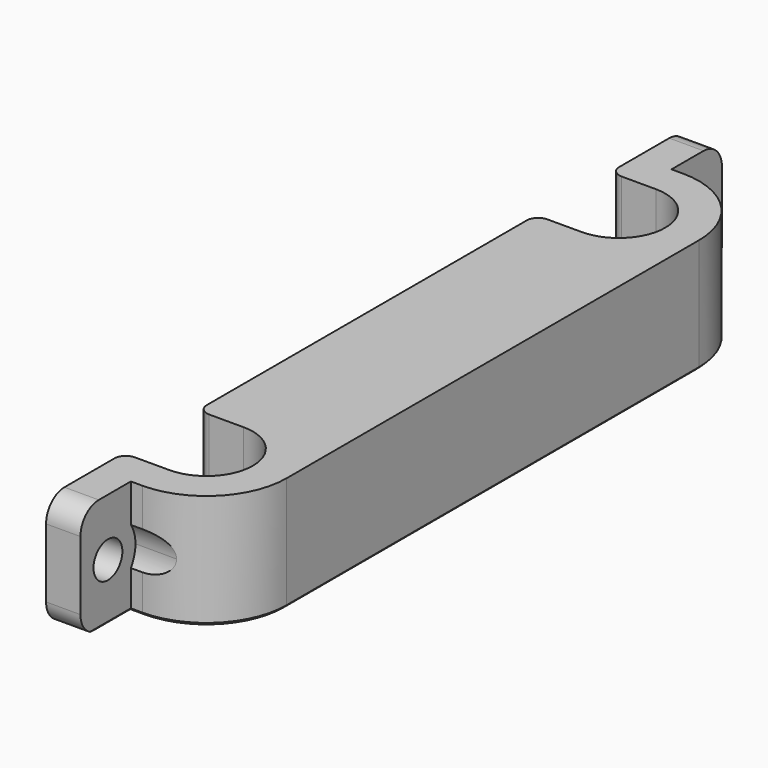
from build123d import *

# Parameters (mm, degrees)
F1_DEPTH     = 5
F2_R         = 1
F3_R         = 1.575
F4_DEPTH     = 3
F3_R_2       = 3
F5_DEPTH     = 8.001
F6_R         = 2
F7_T1_DEPTH  = 6.5429652699
F7_T3_DEPTH  = 3
F7_T5_DEPTH  = 45
F7_T7_DEPTH  = 34.9
F7_T9_DEPTH  = 6.5429652699
F7_T12_ANGLE = 90
F7_T16_DEPTH = 5.2358860169
F7_T21_DEPTH = 1.642920747
F7_T24_ANGLE = 180
F7_T26_ANGLE = 90
F7_T28_ANGLE = 90
F7_T30_ANGLE = 90
F7_T34_DEPTH = 1.642920747
F7_T37_ANGLE = 90
F7_T41_DEPTH = 5.2358860169
F7_T44_ANGLE = 180
F7_T46_ANGLE = 90


# Not quite as in the source:
# - a fillet or chamfer that OpenCascade refuses, or shapes differently, is made with other operations: its cross-section is extruded or revolved along the edge and cut away or added


with BuildPart() as f1:
    # F0 (on Top) → F1 (new body, symmetric)
    with BuildSketch(Plane.XY):
        with BuildLine():
            Line((-4, 26.55), (0, 26.55))
            ThreePointArc((0, 26.55), (4.05, 22.5), (0, 18.45))
            Line((0, 18.45), (-4, 18.45))
            Line((-4, 18.45), (-4, 0))
            Line((-4, 0), (-4, -18.45))
            Line((-4, -18.45), (0, -18.45))
            ThreePointArc((0, -18.45), (4.05, -22.5), (0, -26.55))
            Line((0, -26.55), (-4, -26.55))
            Line((-4, -26.55), (-4, -35))
            Line((-4, -35), (-1, -35))
            Line((-1, -35), (-1, -29.5))
            Line((-1, -29.5), (0, -29.5))
            ThreePointArc((0, -29.5), (4.9497474683, -27.4497474683), (7, -22.5))
            Line((7, -22.5), (7, 0))
            Line((7, 0), (7, 22.5))
            ThreePointArc((7, 22.5), (4.9497474683, 27.4497474683), (0, 29.5))
            Line((0, 29.5), (-1, 29.5))
            Line((-1, 29.5), (-1, 35))
            Line((-1, 35), (-4, 35))
            Line((-4, 35), (-4, 26.55))
        make_face()
    extrude(amount=F1_DEPTH, both=True)

    # F2
    f2_edges = [f1.edges().sort_by_distance(p)[0] for p in [
        (-4, 26.55, 0),
        (-4, 18.45, 0),
        (-4, -26.55, 0),
        (-4, -18.45, 0),
    ]]
    fillet(f2_edges, radius=F2_R)

    # F3 (on face) → F4 (cut, through all)
    with BuildSketch(Plane.YZ.offset(-1)):
        with Locations((32, 0)):
            Circle(F3_R)
        with Locations((-32, 0)):
            Circle(F3_R)
    extrude(amount=-F4_DEPTH, mode=Mode.SUBTRACT)

    # F3 (on face) → F5 (cut, through all)
    with BuildSketch(Plane.YZ.offset(-1)):
        with Locations((32, 0)):
            Circle(F3_R_2)
        with Locations((32, 0)):
            Circle(F3_R, mode=Mode.SUBTRACT)
        with BuildLine():
            ThreePointArc((-29.5, -1.6583123952), (-29.1277186767, -0.8660254038), (-29, 0))
            ThreePointArc((-29, 0), (-29.1277186767, 0.8660254038), (-29.5, 1.6583123952))
            Line((-29.5, 1.6583123952), (-29.5, -1.6583123952))
        make_face()
        with BuildLine():
            Line((-29.5, -1.6583123952), (-29.5, 1.6583123952))
            ThreePointArc((-29.5, 1.6583123952), (-32.8660254038, 2.8722813233), (-35, 0))
            ThreePointArc((-35, 0), (-32.8660254038, -2.8722813233), (-29.5, -1.6583123952))
        make_face()
        with Locations((-32, 0)):
            Circle(F3_R, mode=Mode.SUBTRACT)
    extrude(amount=F5_DEPTH, mode=Mode.SUBTRACT)

    # F6
    f6_edges = [f1.edges().sort_by_distance(p)[0] for p in [
        (-2.5, 35, -5),
        (-2.5, 35, 5),
        (-2.5, -35, -5),
        (-2.5, -35, 5),
    ]]
    fillet(f6_edges, radius=F6_R)

    # F7: chamfer of 0.25 on 22 edges, made by hand

    # F7_s2 → F7_t1 (cut)
    with BuildSketch(Plane.XZ.offset(-34.0929652699)):
        Polygon((-3.75, -5), (-4, -4.75), (-4, -5), align=None)
    extrude(amount=F7_T1_DEPTH, mode=Mode.SUBTRACT)

    # F7_s4 → F7_t3 (cut)
    with BuildSketch(Plane.YZ.offset(-3)):
        Polygon((26.8, -5), (26.55, -4.75), (26.55, -5), align=None)
        Polygon((18.2, -5), (18.45, -4.75), (18.45, -5), align=None)
        Polygon((-18.2, -5), (-18.45, -4.75), (-18.45, -5), align=None)
        Polygon((-26.8, -5), (-26.55, -4.75), (-26.55, -5), align=None)
    extrude(amount=F7_T3_DEPTH, mode=Mode.SUBTRACT)

    # F7_s6 → F7_t5 (cut)
    with BuildSketch(Plane.XZ.offset(-22.5)):
        Polygon((6.75, -5), (7, -4.75), (7, -5), align=None)
    extrude(amount=F7_T5_DEPTH, mode=Mode.SUBTRACT)

    # F7_s8 → F7_t7 (cut)
    with BuildSketch(Plane.XZ.offset(-17.45)):
        Polygon((-3.75, -5), (-4, -4.75), (-4, -5), align=None)
    extrude(amount=F7_T7_DEPTH, mode=Mode.SUBTRACT)

    # F7_s10 → F7_t9 (cut)
    with BuildSketch(Plane.XZ.offset(27.55)):
        Polygon((-4, -4.75), (-3.75, -5), (-4, -5), align=None)
    extrude(amount=F7_T9_DEPTH, mode=Mode.SUBTRACT)

    # F7_s11 → F7_t12 (revolve, cut)
    with BuildSketch(Plane.YZ.offset(-3)):
        Polygon((26.8, -5), (26.55, -4.75), (26.55, -5), align=None)
    revolve(axis=Axis((-3, 27.55, -5), (0, 0, -1)), revolution_arc=F7_T12_ANGLE, mode=Mode.SUBTRACT)


with BuildPart() as f7_tool14:
    # F7_s15 → F7_t16 (new body)
    with BuildSketch(Plane.XZ.offset(-28.857079253)):
        Polygon((-1.25, -5), (-1, -4.75), (-1, -5), align=None)
    extrude(amount=-F7_T16_DEPTH)

    split(bisect_by=Plane(origin=(0, 17.125, -17.125), x_dir=(1, 0, 0), z_dir=(0, 0.7071067812, -0.7071067812)), keep=Keep.TOP)


with BuildPart() as f1_1:
    add(f1.part)

    # F7_t13: cut F7_tool14
    add(f7_tool14.part, mode=Mode.SUBTRACT)


with BuildPart() as f7_tool19:
    # F7_s20 → F7_t21 (new body)
    with BuildSketch(Plane.YZ):
        Polygon((29.25, -5), (29.5, -4.75), (29.5, -5), align=None)
    extrude(amount=-F7_T21_DEPTH)

    split(bisect_by=Plane(origin=(1.875, 0, -1.875), x_dir=(0, 1, 0), z_dir=(0.7071067812, 0, -0.7071067812)), keep=Keep.TOP)


with BuildPart() as f1_2:
    add(f1_1.part)

    # F7_t18: cut F7_tool19
    add(f7_tool19.part, mode=Mode.SUBTRACT)

    # F7_s23 → F7_t24 (revolve, cut)
    with BuildSketch(Plane.YZ):
        Polygon((26.8, -5), (26.55, -4.75), (26.55, -5), align=None)
    revolve(axis=Axis((0, 22.5, -5), (0, 0, -1)), revolution_arc=F7_T24_ANGLE, mode=Mode.SUBTRACT)

    # F7_s25 → F7_t26 (revolve, cut)
    with BuildSketch(Plane.XZ.offset(-22.5)):
        Polygon((6.75, -5), (7, -4.75), (7, -5), align=None)
    revolve(axis=Axis((0, 22.5, -5), (0, 0, 1)), revolution_arc=F7_T26_ANGLE, mode=Mode.SUBTRACT)

    # F7_s27 → F7_t28 (revolve, cut)
    with BuildSketch(Plane.XZ.offset(-17.45)):
        Polygon((-3.75, -5), (-4, -4.75), (-4, -5), align=None)
    revolve(axis=Axis((-3, 17.45, -5), (0, 0, -1)), revolution_arc=F7_T28_ANGLE, mode=Mode.SUBTRACT)

    # F7_s29 → F7_t30 (revolve, cut)
    with BuildSketch(Plane.YZ):
        Polygon((-29.25, -5), (-29.5, -4.75), (-29.5, -5), align=None)
    revolve(axis=Axis((0, -22.5, -5), (0, 0, 1)), revolution_arc=F7_T30_ANGLE, mode=Mode.SUBTRACT)


with BuildPart() as f7_tool32:
    # F7_s33 → F7_t34 (new body)
    with BuildSketch(Plane.YZ.offset(-1.642920747)):
        Polygon((-29.25, -5), (-29.5, -4.75), (-29.5, -5), align=None)
    extrude(amount=F7_T34_DEPTH)

    split(bisect_by=Plane(origin=(1.875, 0, -1.875), x_dir=(0, 1, 0), z_dir=(0.7071067812, 0, -0.7071067812)), keep=Keep.TOP)


with BuildPart() as f1_3:
    add(f1_2.part)

    # F7_t31: cut F7_tool32
    add(f7_tool32.part, mode=Mode.SUBTRACT)

    # F7_s36 → F7_t37 (revolve, cut)
    with BuildSketch(Plane.YZ.offset(-3)):
        Polygon((-18.2, -5), (-18.45, -4.75), (-18.45, -5), align=None)
    revolve(axis=Axis((-3, -17.45, -5), (0, 0, -1)), revolution_arc=F7_T37_ANGLE, mode=Mode.SUBTRACT)


with BuildPart() as f7_tool39:
    # F7_s40 → F7_t41 (new body)
    with BuildSketch(Plane.XZ.offset(34.0929652699)):
        Polygon((-1.25, -5), (-1, -4.75), (-1, -5), align=None)
    extrude(amount=-F7_T41_DEPTH)

    split(bisect_by=Plane(origin=(0, -17.125, -17.125), x_dir=(1, 0, 0), z_dir=(0, -0.7071067812, -0.7071067812)), keep=Keep.TOP)


with BuildPart() as f1_4:
    add(f1_3.part)

    # F7_t38: cut F7_tool39
    add(f7_tool39.part, mode=Mode.SUBTRACT)

    # F7_s43 → F7_t44 (revolve, cut)
    with BuildSketch(Plane.YZ):
        Polygon((-18.2, -5), (-18.45, -4.75), (-18.45, -5), align=None)
    revolve(axis=Axis((0, -22.5, -5), (0, 0, -1)), revolution_arc=F7_T44_ANGLE, mode=Mode.SUBTRACT)

    # F7_s45 → F7_t46 (revolve, cut)
    with BuildSketch(Plane.XZ.offset(27.55)):
        Polygon((-3.75, -5), (-4, -4.75), (-4, -5), align=None)
    revolve(axis=Axis((-3, -27.55, -5), (0, 0, -1)), revolution_arc=F7_T46_ANGLE, mode=Mode.SUBTRACT)


solid = f1_4.part
